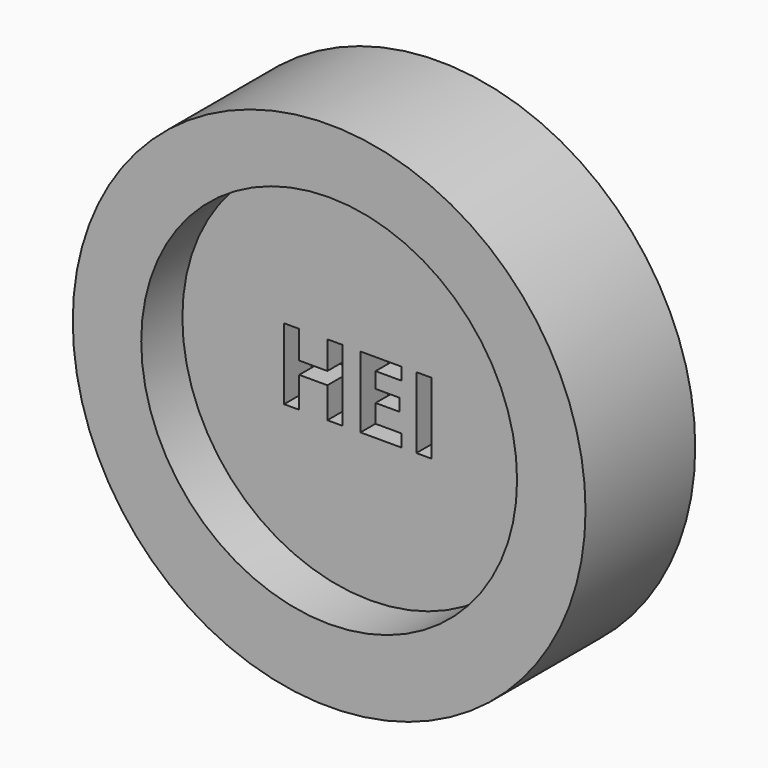
from build123d import *

# Parameters (mm, degrees)
F0_R         = 74.7863205326
F1_DEPTH     = 25
F2_TEXT_SIZE = 29.1142108229
F3_DEPTH     = 10
F4_R         = 74.7863205326
F4_R_2       = 54.8130928287
F5_DEPTH     = 15


# Not quite as in the source:
# - Text() gives the source's letters only with a copy of the font that has no kerning and outlines rounded to 1/6400 em; it was checked with that copy


with BuildPart() as f1:
    # F0 (on Front) → F1 (new body)
    with BuildSketch(Plane.XZ):
        Circle(F0_R)
    extrude(amount=F1_DEPTH)

    # F2 (on face) → F3 (cut)
    with BuildSketch(Plane.XZ.offset(25)):
        with Locations((-27.7607925236, -11.3309361041)):
            Text('HEI', F2_TEXT_SIZE, font='Open Sans', font_style=FontStyle.BOLD, text_align=(TextAlign.LEFT, TextAlign.BOTTOM))
    extrude(amount=-F3_DEPTH, mode=Mode.SUBTRACT)

    # F4 (on face) → F5 (join)
    with BuildSketch(Plane.XZ.offset(25)):
        Circle(F4_R)
        with Locations((0, 1.2791564586)):
            Circle(F4_R_2, mode=Mode.SUBTRACT)
    extrude(amount=F5_DEPTH)


solid = f1.part
